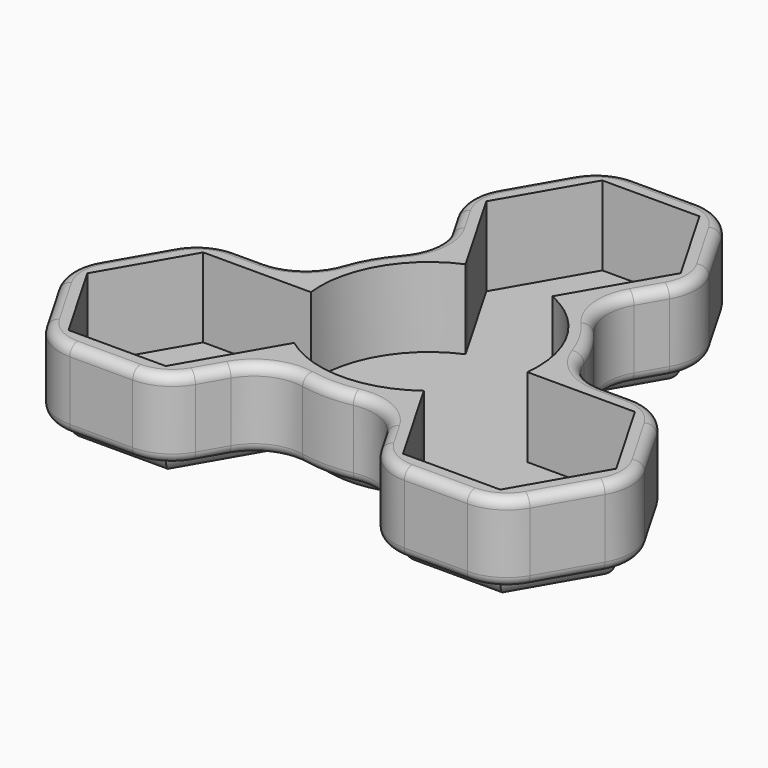
from build123d import *

# Parameters (mm, degrees)
F1_DEPTH = 8
F2_R     = 5
F3_R     = 5
F4_R     = 1
F5_DEPTH = 2
F6_R     = 1.99999


# Not quite as in the source:
# - a fillet or chamfer is up to 0.001 mm smaller than in the source, because OpenCascade refuses the exact size


with BuildPart() as f1:
    # F0 (on Top) → F1 (new body)
    with BuildSketch(Plane.XY):
        with BuildLine():
            Line((6.0621778265, 30), (-6.0621778265, 30))
            Line((-6.0621778265, 30), (-12.124355653, 19.5))
            Line((-12.124355653, 19.5), (-7.138692729, 10.8645785063))
            ThreePointArc((-7.138692729, 10.8645785063), (-11.2583302492, 6.5), (-12.9783473524, 0.75))
            Line((-12.9783473524, 0.75), (-22.9496732003, 0.75))
            Line((-22.9496732003, 0.75), (-29.0118510268, -9.75))
            Line((-29.0118510268, -9.75), (-22.9496732003, -20.25))
            Line((-22.9496732003, -20.25), (-10.8253175473, -20.25))
            Line((-10.8253175473, -20.25), (-5.8396546234, -11.6145785063))
            ThreePointArc((-5.8396546234, -11.6145785063), (0, -13), (5.8396546234, -11.6145785063))
            Line((5.8396546234, -11.6145785063), (10.8253175473, -20.25))
            Line((10.8253175473, -20.25), (22.9496732003, -20.25))
            Line((22.9496732003, -20.25), (29.0118510268, -9.75))
            Line((29.0118510268, -9.75), (22.9496732003, 0.75))
            Line((22.9496732003, 0.75), (12.9783473524, 0.75))
            ThreePointArc((12.9783473524, 0.75), (11.2583302492, 6.5), (7.138692729, 10.8645785063))
            Line((7.138692729, 10.8645785063), (12.124355653, 19.5))
            Line((12.124355653, 19.5), (6.0621778265, 30))
        make_face()
        with BuildLine():
            Line((-9.8149545762, 19.5), (-4.9074772881, 28))
            Line((-4.9074772881, 28), (4.9074772881, 28))
            Line((4.9074772881, 28), (9.8149545762, 19.5))
            Line((9.8149545762, 19.5), (4.9074772881, 11))
            Line((4.9074772881, 11), (4.3818414939, 10.0895720981))
            ThreePointArc((4.3818414939, 10.0895720981), (9.5262794416, 5.5), (10.9287464972, -1.25))
            Line((10.9287464972, -1.25), (11.9800180857, -1.25))
            Line((11.9800180857, -1.25), (21.7949726619, -1.25))
            Line((21.7949726619, -1.25), (26.70244995, -9.75))
            Line((26.70244995, -9.75), (21.7949726619, -18.25))
            Line((21.7949726619, -18.25), (11.9800180857, -18.25))
            Line((11.9800180857, -18.25), (7.0725407976, -9.75))
            Line((7.0725407976, -9.75), (6.5469050033, -8.8395720981))
            ThreePointArc((6.5469050033, -8.8395720981), (0, -11), (-6.5469050033, -8.8395720981))
            Line((-6.5469050033, -8.8395720981), (-7.0725407976, -9.75))
            Line((-7.0725407976, -9.75), (-11.9800180857, -18.25))
            Line((-11.9800180857, -18.25), (-21.7949726619, -18.25))
            Line((-21.7949726619, -18.25), (-26.70244995, -9.75))
            Line((-26.70244995, -9.75), (-21.7949726619, -1.25))
            Line((-21.7949726619, -1.25), (-11.9800180857, -1.25))
            Line((-11.9800180857, -1.25), (-10.9287464972, -1.25))
            ThreePointArc((-10.9287464972, -1.25), (-9.5262794416, 5.5), (-4.3818414939, 10.0895720981))
            Line((-4.3818414939, 10.0895720981), (-4.9074772881, 11))
            Line((-4.9074772881, 11), (-9.8149545762, 19.5))
        make_face(mode=Mode.SUBTRACT)
    extrude(amount=F1_DEPTH)

    # F2
    f2_edges = [f1.edges().sort_by_distance(p)[0] for p in [
        (12.978347, 0.75, 4),
        (7.138693, 10.864579, 4),
        (5.839655, -11.614579, 4),
        (-5.839655, -11.614579, 4),
        (-12.978347, 0.75, 4),
        (-7.138693, 10.864579, 4),
    ]]
    fillet(f2_edges, radius=F2_R)

    # F3
    f3_edges = [f1.edges().sort_by_distance(p)[0] for p in [
        (10.825318, -20.25, 4),
        (22.949673, -20.25, 4),
        (29.011851, -9.75, 4),
        (22.949673, 0.75, 4),
        (12.124356, 19.5, 4),
        (6.062178, 30, 4),
        (-6.062178, 30, 4),
        (-12.124356, 19.5, 4),
        (-22.949673, 0.75, 4),
        (-29.011851, -9.75, 4),
        (-22.949673, -20.25, 4),
        (-10.825318, -20.25, 4),
    ]]
    fillet(f3_edges, radius=F3_R)

    # F4
    f4_edges = [f1.edges().sort_by_distance(p)[0] for p in [
        (25.980762, -15, 8),
        (22.562922, -19.580127, 8),
        (16.887495, -20.25, 8),
        (11.212069, -19.580127, 8),
        (8.630434, -16.44835, 8),
        (5.607537, -13.090211, 8),
        (0, -13, 8),
        (-5.607537, -13.090211, 8),
        (-11.212069, -19.580127, 8),
        (-8.630434, -16.44835, 8),
        (-16.887495, -20.25, 8),
        (-22.562922, -19.580127, 8),
        (-25.980762, -15, 8),
        (-28.238348, -9.75, 8),
        (-25.980762, -4.5, 8),
        (-22.562922, 0.080127, 8),
        (-18.559906, 0.75, 8),
        (-14.140223, 1.688836, 8),
        (-8.532686, 11.401375, 8),
        (-11.25833, 6.5, 8),
        (-9.929472, 15.69835, 8),
        (-11.350853, 19.5, 8),
        (-9.093267, 24.75, 8),
        (-5.675426, 29.330127, 8),
        (0, 30, 8),
        (5.675426, 29.330127, 8),
        (9.093267, 24.75, 8),
        (11.350853, 19.5, 8),
        (9.929472, 15.69835, 8),
        (8.532686, 11.401375, 8),
        (11.25833, 6.5, 8),
        (14.140223, 1.688836, 8),
        (18.559906, 0.75, 8),
        (22.562922, 0.080127, 8),
        (25.980762, -4.5, 8),
        (28.238348, -9.75, 8),
        (-25.980762, -4.5, 0),
        (-28.238348, -9.75, 0),
        (-25.980762, -15, 0),
        (-22.562922, -19.580127, 0),
    ]]
    fillet(f4_edges, radius=F4_R)


with BuildPart() as f5:
    # F0 (on Top) → F5 (new body)
    with BuildSketch(Plane.XY):
        with BuildLine():
            Line((4.9074772881, 28), (-4.9074772881, 28))
            Line((-4.9074772881, 28), (-9.8149545762, 19.5))
            Line((-9.8149545762, 19.5), (-4.9074772881, 11))
            Line((-4.9074772881, 11), (-4.3818414939, 10.0895720981))
            ThreePointArc((-4.3818414939, 10.0895720981), (-9.5262794416, 5.5), (-10.9287464972, -1.25))
            Line((-10.9287464972, -1.25), (-11.9800180857, -1.25))
            Line((-11.9800180857, -1.25), (-21.7949726619, -1.25))
            Line((-21.7949726619, -1.25), (-26.70244995, -9.75))
            Line((-26.70244995, -9.75), (-21.7949726619, -18.25))
            Line((-21.7949726619, -18.25), (-11.9800180857, -18.25))
            Line((-11.9800180857, -18.25), (-7.0725407976, -9.75))
            Line((-7.0725407976, -9.75), (-6.5469050033, -8.8395720981))
            ThreePointArc((-6.5469050033, -8.8395720981), (0, -11), (6.5469050033, -8.8395720981))
            Line((6.5469050033, -8.8395720981), (7.0725407976, -9.75))
            Line((7.0725407976, -9.75), (11.9800180857, -18.25))
            Line((11.9800180857, -18.25), (21.7949726619, -18.25))
            Line((21.7949726619, -18.25), (26.70244995, -9.75))
            Line((26.70244995, -9.75), (21.7949726619, -1.25))
            Line((21.7949726619, -1.25), (11.9800180857, -1.25))
            Line((11.9800180857, -1.25), (10.9287464972, -1.25))
            ThreePointArc((10.9287464972, -1.25), (9.5262794416, 5.5), (4.3818414939, 10.0895720981))
            Line((4.3818414939, 10.0895720981), (4.9074772881, 11))
            Line((4.9074772881, 11), (9.8149545762, 19.5))
            Line((9.8149545762, 19.5), (4.9074772881, 28))
        make_face()
    extrude(amount=-F5_DEPTH)

    # F6 (radius 2 in the source; OpenCascade refuses exactly that, so slightly less here)
    f6_edges = [f5.edges().sort_by_distance(p)[0] for p in [
        (7.361216, 23.75, -2),
        (0, 28, -2),
        (-7.361216, 23.75, -2),
        (-7.098398, 14.794786, -2),
        (-9.526279, 5.5, -2),
        (-16.36186, -1.25, -2),
        (-24.248711, -5.5, -2),
        (-24.248711, -14, -2),
        (-16.887495, -18.25, -2),
        (-9.263462, -13.544786, -2),
        (0, -11, -2),
        (9.263462, -13.544786, -2),
        (16.887495, -18.25, -2),
        (24.248711, -14, -2),
        (24.248711, -5.5, -2),
        (16.36186, -1.25, -2),
        (9.526279, 5.5, -2),
        (7.098398, 14.794786, -2),
    ]]
    fillet(f6_edges, radius=F6_R)


solid = Compound([f1.part, f5.part])
